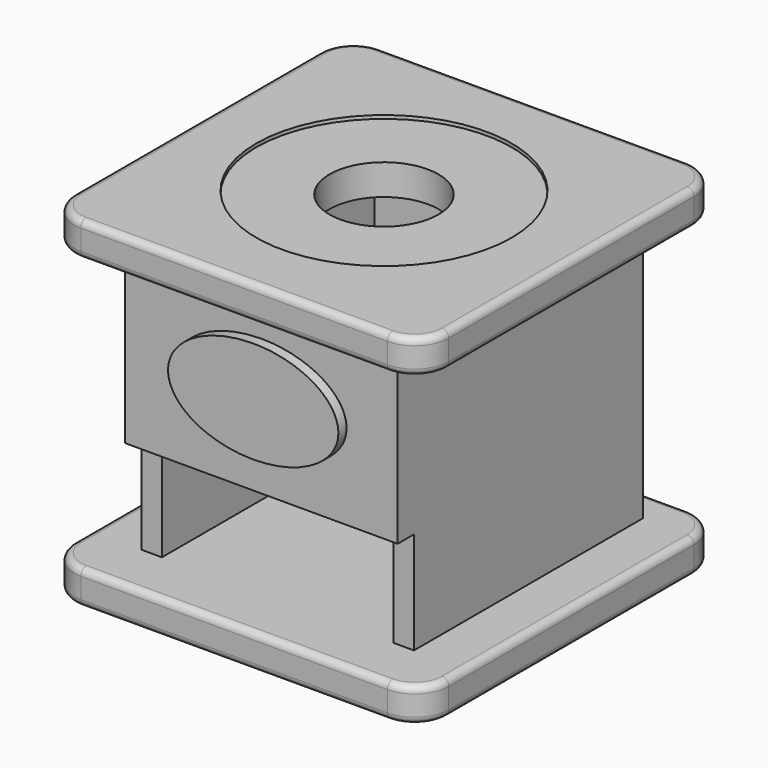
from build123d import *

# Parameters (mm, degrees)
F0_W            = 80
F0_H            = 90
F1_DEPTH        = 50
F2_W            = 68
F2_H            = 78
F3_DEPTH        = 50.001
F3_DEPTH_BACK   = 50.001
F4_W            = 110
F4_H            = 110
F5_DEPTH        = 10
F5_COPIES_COUNT = 2
F5_COPIES_PITCH = 90
F6_R            = 10
F7_R            = 2
F8_W            = 80
F8_H            = 30
F9_DEPTH        = 6
F10_R           = 37.5
F11_DEPTH       = 1
F12_R           = 16
F13_DEPTH       = 9
F15_DEPTH       = 3


# Not quite as in the source:
# - a pattern or mirror of a feature is missing from the dataset's text; its kind, count and spacing are read off the source's solid


with BuildPart() as f1:
    # F0 (on Top) → F1 (new body, symmetric)
    with BuildSketch(Plane.XY):
        Rectangle(F0_W, F0_H)
    extrude(amount=F1_DEPTH, both=True)

    # F2 (on Top) → F3 (cut, two sides)
    with BuildSketch(Plane.XY) as f3_sk:
        Rectangle(F2_W, F2_H)
    extrude(amount=-F3_DEPTH, mode=Mode.SUBTRACT)
    extrude(f3_sk.sketch, amount=F3_DEPTH_BACK, mode=Mode.SUBTRACT)

    # F4 (on face) → F5 (join)
    with BuildSketch(Plane(origin=(0, 0, -50), x_dir=(1, 0, 0), z_dir=(0, 0, -1))):
        Rectangle(F4_W, F4_H)
    f5 = extrude(amount=-F5_DEPTH)

    # F5_copies: F5 ×2
    with Locations(*[(0, 0, i * F5_COPIES_PITCH) for i in range(1, F5_COPIES_COUNT)]):
        add(f5)

    # F6
    f6_edges = [f1.edges().sort_by_distance(p)[0] for p in [
        (55, -55, -45),
        (55, 55, -45),
        (-55, -55, -45),
        (-55, 55, -45),
        (55, 55, 45),
        (55, -55, 45),
        (-55, 55, 45),
        (-55, -55, 45),
    ]]
    fillet(f6_edges, radius=F6_R)

    # F7
    f7_edges = [f1.edges().sort_by_distance(p)[0] for p in [
        (0, -55, -40),
        (0, -55, -50),
        (55, 0, -50),
        (52.071068, 52.071068, -50),
        (52.071068, -52.071068, -50),
        (0, 55, -50),
        (-52.071068, 52.071068, -50),
        (-52.071068, -52.071068, -50),
        (-55, 0, -50),
        (55, 0, -40),
        (52.071068, 52.071068, -40),
        (52.071068, -52.071068, -40),
        (0, 55, -40),
        (-52.071068, 52.071068, -40),
        (-52.071068, -52.071068, -40),
        (-55, 0, -40),
        (55, 0, 40),
        (52.071068, 52.071068, 40),
        (52.071068, -52.071068, 40),
        (0, 55, 40),
        (0, -55, 40),
        (-52.071068, 52.071068, 40),
        (-52.071068, -52.071068, 40),
        (-55, 0, 40),
        (55, 0, 50),
        (52.071068, 52.071068, 50),
        (52.071068, -52.071068, 50),
        (0, 55, 50),
        (0, -55, 50),
        (-52.071068, 52.071068, 50),
        (-52.071068, -52.071068, 50),
        (-55, 0, 50),
    ]]
    fillet(f7_edges, radius=F7_R)

    # F8 (on face) → F9 (cut)
    with BuildSketch(Plane.XZ.offset(45)):
        with Locations((0, -25)):
            Rectangle(F8_W, F8_H)
    extrude(amount=-F9_DEPTH, mode=Mode.SUBTRACT)

    # F10 (on face) → F11 (cut)
    with BuildSketch(Plane.XY.offset(50)):
        Circle(F10_R)
    extrude(amount=-F11_DEPTH, mode=Mode.SUBTRACT)

    # F12 (on face) → F13 (cut, through all)
    with BuildSketch(Plane.XY.offset(49)):
        Circle(F12_R)
    extrude(amount=-F13_DEPTH, mode=Mode.SUBTRACT)

    # F14 (on face) → F15 (join)
    with BuildSketch(Plane.XZ.offset(45)):
        with BuildLine():
            add(Edge.make_bspline(
                [(0, 30), (-43.3012701892, 30), (-21.6506350946, 7.5), (0, -15), (21.6506350946, 7.5), (43.3012701892, 30), (0, 30)],
                knots=[4.7123889804, 4.7123889804, 4.7123889804, 6.8067840828, 6.8067840828, 8.9011791852, 8.9011791852, 10.9955742876, 10.9955742876, 10.9955742876], degree=2, weights=[1, 0.5, 1, 0.5, 1, 0.5, 1]))
        make_face()
    extrude(amount=F15_DEPTH)


solid = f1.part
